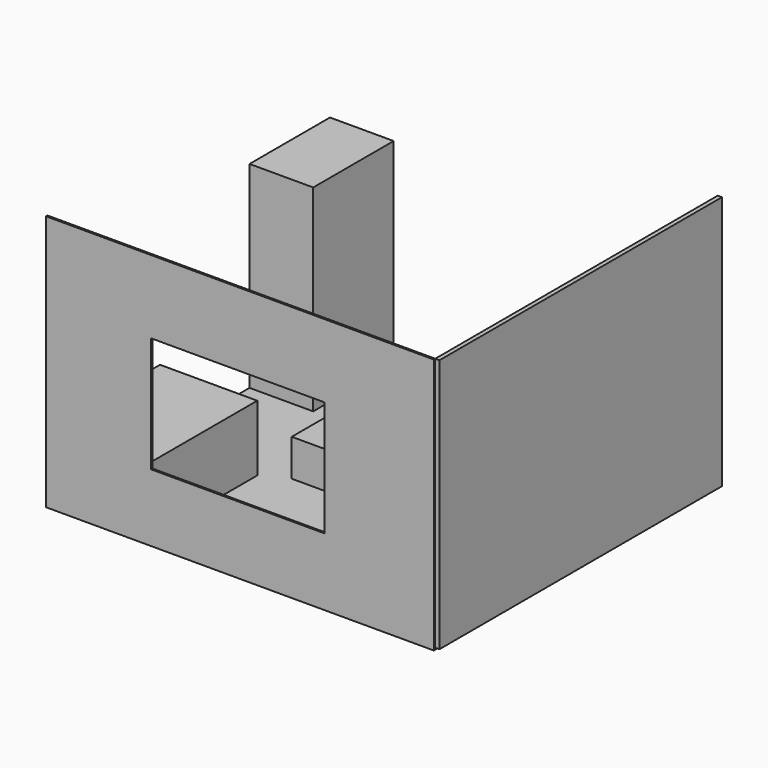
from build123d import *

# Parameters (mm, degrees)
F0_W        = 5600
F0_H        = 5100
F2_DEPTH    = 25.4
F6_E3_W     = 1550
F6_E3_H     = 750
F7_DEPTH    = 30
F8_W        = 750
F8_H        = 30
F9_DEPTH    = 1550
F1_E0_TOP_W = 5600
F1_E0_TOP_H = 3700
F10_DEPTH   = 25.4
F4_E1_W     = 5100
F4_E1_H     = 3674.5926
F11_DEPTH   = 60.96
F12_W       = 2505.4972171783
F12_H       = 1666.2773489952
F13_DEPTH   = 330.2
F14_W       = 1404.4142246246
F14_H       = 975.7207036018
F15_DEPTH   = 2032
F16_W       = 919.6570396423
F16_H       = 1452.5243520737
F17_DEPTH   = 2847.34
F18_W       = 2083.2133293152
F18_H       = 676.1979460716
F19_DEPTH   = 533.4
F20_W       = 1535.2616906166
F20_H       = 313.4592056274
F21_DEPTH   = 304.8


with BuildPart() as f2:
    # F0 (on Top) → F2 (new body)
    with BuildSketch(Plane.XY):
        Rectangle(F0_W, F0_H)
    extrude(amount=F2_DEPTH)


with BuildPart() as f7:
    # F6_E3 (on explicit) → F7 (new body)
    with BuildSketch(Plane(origin=(2800, -2550, 940), x_dir=(-1, 0, 0), z_dir=(0, 0, -1))):
        with Locations((775, 375)):
            Rectangle(F6_E3_W, F6_E3_H)
    extrude(amount=F7_DEPTH)

    # F8 (on face) → F9 (join)
    with BuildSketch(Plane(origin=(0, -1800, 0), x_dir=(-1, 0, 0), z_dir=(0, 1, 0))):
        with Locations((-2425, 925)):
            Rectangle(F8_W, F8_H)
    extrude(amount=F9_DEPTH)


with BuildPart() as f10:
    # F1_E0_top (on explicit) → F10 (new body)
    with BuildSketch(Plane(origin=(2800, -2550, 0), x_dir=(-1, 0, 0), z_dir=(0, 1, 0))):
        with Locations((2800, 1850)):
            Rectangle(F1_E0_TOP_W, F1_E0_TOP_H)
    extrude(amount=-F10_DEPTH)

    # F12 (on face) → F13 (cut)
    with BuildSketch(Plane(origin=(0, -2550, 0), x_dir=(-1, 0, 0), z_dir=(0, 1, 0))):
        with Locations((33.3737134933, 1808.8593780994)):
            Rectangle(F12_W, F12_H)
    extrude(amount=-F13_DEPTH, mode=Mode.SUBTRACT)


with BuildPart() as f11:
    # F4_E1 (on explicit) → F11 (new body)
    with BuildSketch(Plane(origin=(2800, 2550, 25.4), x_dir=(0, -1, 0), z_dir=(-1, 0, 0))):
        with Locations((2550, 1837.2963)):
            Rectangle(F4_E1_W, F4_E1_H)
    extrude(amount=-F11_DEPTH)


with BuildPart() as f15:
    # F14 (on face) → F15 (new body)
    with BuildSketch(Plane(origin=(0, -2550, 0), x_dir=(-1, 0, 0), z_dir=(0, 1, 0))):
        with Locations((2097.7928876877, 487.8603518009)):
            Rectangle(F14_W, F14_H)
    extrude(amount=F15_DEPTH)


with BuildPart() as f17:
    # F16 (on face) → F17 (new body)
    with BuildSketch(Plane.XY.offset(25.4)):
        with Locations((-2340.1714801788, 1823.7378239632)):
            Rectangle(F16_W, F16_H)
    extrude(amount=F17_DEPTH)


with BuildPart() as f19:
    # F18 (on face) → F19 (new body)
    with BuildSketch(Plane.XY.offset(25.4)):
        Rectangle(F18_W, F18_H)
    extrude(amount=F19_DEPTH)


with BuildPart() as f21:
    # F20 (on face) → F21 (new body)
    with BuildSketch(Plane.XY.offset(25.4)):
        with Locations((-72.6961791515, 2393.2703971863)):
            Rectangle(F20_W, F20_H)
    extrude(amount=F21_DEPTH)


solid = Compound([f2.part, f7.part, f10.part, f11.part, f15.part, f17.part, f19.part, f21.part])
